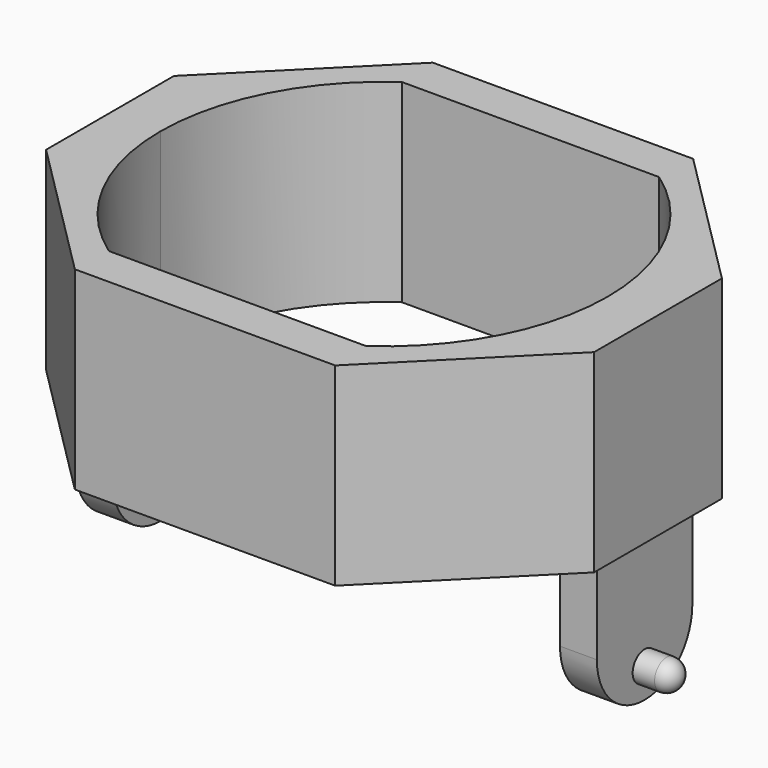
from build123d import *

# Parameters (mm, degrees)
F1_DEPTH  = 16.51
F3_DEPTH  = 6.35
F4_R      = 0.635
F5_DEPTH  = 1.5691231
F6_R      = 2.53999
F7_R      = 0.635
F9_DEPTH  = 6.35
F11_D     = 2.54
F16_D     = 127
F16_DEPTH = 14.606


# Not quite as in the source:
# - a fillet or chamfer is up to 0.001 mm smaller than in the source, because OpenCascade refuses the exact size
# - a length typed as a fraction of an inch, garbled in the dataset ("3 / 203.2 mm" for 3/8 in), is restored
# - the program builds the solid bodies; features that only make, move or delete a surface that nothing else refers to are left out


with BuildPart() as f1:
    # F0 (on Top) → F1 (new body)
    with BuildSketch(Plane.XY):
        Polygon((5.5418181818, 9.525), (0, 9.525), (-5.5418181818, 9.525), (-11.6647200825, 3.4020980993), (-11.6647200825, 0), (-11.6647200825, -3.4020980993), (-5.5418181818, -9.525), (0, -9.525), (5.5418181818, -9.525), (11.6647200825, -3.4020980993), (11.6647200825, 0), (11.6647200825, 3.4020980993), align=None)
        with BuildLine():
            ThreePointArc((5.4764899478, 7.7931818182), (8.4524905132, 4.3910168667), (9.525, 0))
            ThreePointArc((9.525, 0), (8.4524905132, -4.3910168667), (5.4764899478, -7.7931818182))
            Line((5.4764899478, -7.7931818182), (0, -7.7931818182))
            Line((0, -7.7931818182), (-5.4764899478, -7.7931818182))
            ThreePointArc((-5.4764899478, -7.7931818182), (-8.4524905132, -4.3910168667), (-9.525, 0))
            ThreePointArc((-9.525, 0), (-8.4524905132, 4.3910168667), (-5.4764899478, 7.7931818182))
            Line((-5.4764899478, 7.7931818182), (0, 7.7931818182))
            Line((0, 7.7931818182), (5.4764899478, 7.7931818182))
        make_face(mode=Mode.SUBTRACT)
    extrude(amount=F1_DEPTH)

    # F2 (on Top) → F3 (join)
    with BuildSketch(Plane.XY):
        Polygon((11.0941231, -2.54), (11.0941231, 0), (11.0941231, 2.54), (9.525, 2.54), (9.525, 0), (9.525, -2.54), align=None)
    extrude(amount=-F3_DEPTH)

    # F4 (on face) → F5 (join)
    with BuildSketch(Plane.YZ.offset(11.0941231)):
        with Locations((0, -5.08)):
            Circle(F4_R)
    extrude(amount=F5_DEPTH)

    # F6 (radius 2.54 in the source; OpenCascade refuses exactly that, so slightly less here)
    f6_edges = [f1.edges().sort_by_distance(p)[0] for p in [
        (10.309562, -2.54, -6.35),
        (10.309562, 2.54, -6.35),
    ]]
    fillet(f6_edges, radius=F6_R)

    # F7
    f7_edges = [f1.edges().sort_by_distance(p)[0] for p in [
        (12.663246, -0.635, -5.08),
    ]]
    fillet(f7_edges, radius=F7_R)

    # F8 (on face) → F9 (join)
    with BuildSketch(Plane.XY.offset(16.51)):
        Polygon((11.6647200825, 2.54), (10.095592022, 2.54), (10.095592022, 0), (10.095592022, -2.54), (11.6647200825, -2.54), (11.6647200825, 0), align=None)
    extrude(amount=F9_DEPTH)

    # F11 (through all)
    with Locations(Plane.YZ.offset(11.6647200825)):
        with Locations((0, 20.32)):
            Hole(F11_D / 2)

    # F12: F1 across plane


with BuildPart() as f1_1:
    add(f1.part)
    add(f1.part.mirror(Plane.YZ))

    # F16 (through all, one way)
    with BuildSketch(Plane(origin=(0, 0, 8.255), x_dir=(1, 0, 0), z_dir=(0, 0, -1))):
        with Locations((0, 0)):
            Circle(F16_D / 2)
    extrude(amount=-F16_DEPTH, mode=Mode.SUBTRACT)


solid = f1_1.part
